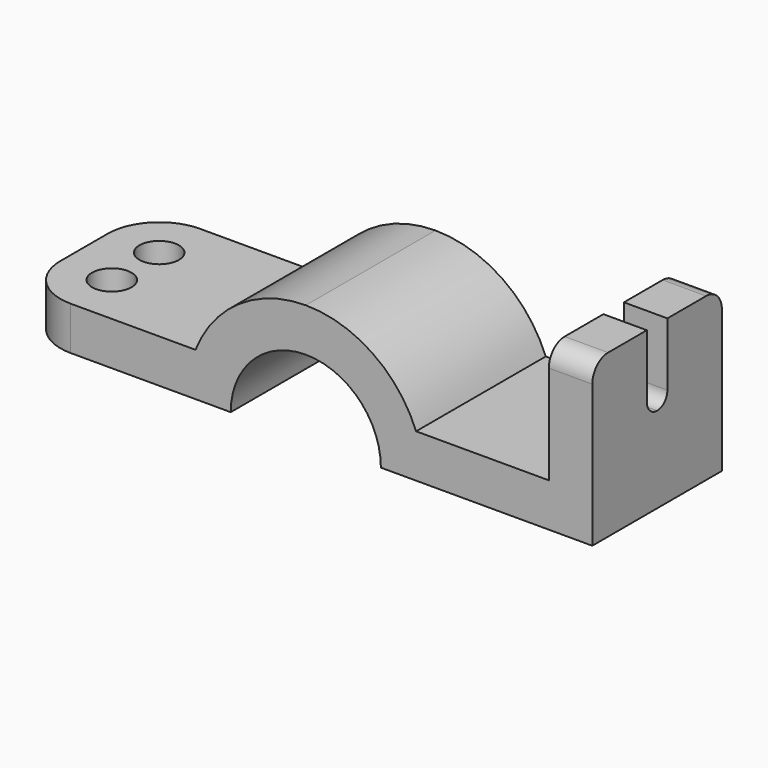
from build123d import *

# Parameters (mm, degrees)
F1_DEPTH = 52.07
F2_R     = 33.02
F3_R     = 12.7
F4_DEPTH = 27.94
F6_DEPTH = 27.94
F7_R     = 12.7


# Not quite as in the source:
# - a pattern or mirror of a feature is missing from the dataset's text; its kind, count and spacing are read off the source's solid


with BuildPart() as f1:
    # F0 (on Front) → F1 (new body, symmetric)
    with BuildSketch(Plane.XZ):
        with BuildLine():
            Line((-184.15, 27.94), (-184.15, 0))
            Line((-184.15, 0), (-48.26, 0))
            ThreePointArc((-48.26, 0), (-34.1249732601, 34.1249732601), (0, 48.26))
            ThreePointArc((0, 48.26), (34.1249732601, 34.1249732601), (48.26, 0))
            Line((48.26, 0), (184.15, 0))
            Line((184.15, 0), (184.15, 104.14))
            Line((184.15, 104.14), (156.21, 104.14))
            Line((156.21, 104.14), (156.21, 27.94))
            Line((156.21, 27.94), (70.8928515437, 27.94))
            ThreePointArc((70.8928515437, 27.94), (42.880135261, 62.9899515796), (0, 76.2))
            ThreePointArc((0, 76.2), (-42.880135261, 62.9899515796), (-70.8928515437, 27.94))
            Line((-70.8928515437, 27.94), (-184.15, 27.94))
        make_face()
    extrude(amount=F1_DEPTH, both=True)

    # F2
    f2_edges = [f1.edges().sort_by_distance(p)[0] for p in [
        (-184.15, 52.07, 13.97),
        (-184.15, -52.07, 13.97),
    ]]
    fillet(f2_edges, radius=F2_R)

    # F3 (on face) → F4 (cut)
    with BuildSketch(Plane.XY.offset(27.94)):
        with Locations((-151.13, 19.05)):
            Circle(F3_R)
        with Locations((-151.13, -19.05)):
            Circle(F3_R)
    extrude(amount=-F4_DEPTH, mode=Mode.SUBTRACT)

    # F5 (on face) → F6 (cut)
    with BuildSketch(Plane.YZ.offset(184.15)):
        with BuildLine():
            Line((0, 104.14), (0, 55.245))
            ThreePointArc((0, 55.245), (5.8371664787, 57.6628335213), (8.255, 63.5))
            Line((8.255, 63.5), (8.255, 104.14))
            Line((8.255, 104.14), (0, 104.14))
        make_face()
    f6 = extrude(amount=-F6_DEPTH, mode=Mode.SUBTRACT)

    # F6_copies: F6 across plane
    add(f6.mirror(Plane(origin=(0, 0, 0), x_dir=(0, 0, -1), z_dir=(0, -1, 0))), mode=Mode.SUBTRACT)

    # F7
    f7_edges = [f1.edges().sort_by_distance(p)[0] for p in [
        (170.18, -52.07, 104.14),
        (170.18, 52.07, 104.14),
    ]]
    fillet(f7_edges, radius=F7_R)


solid = f1.part
